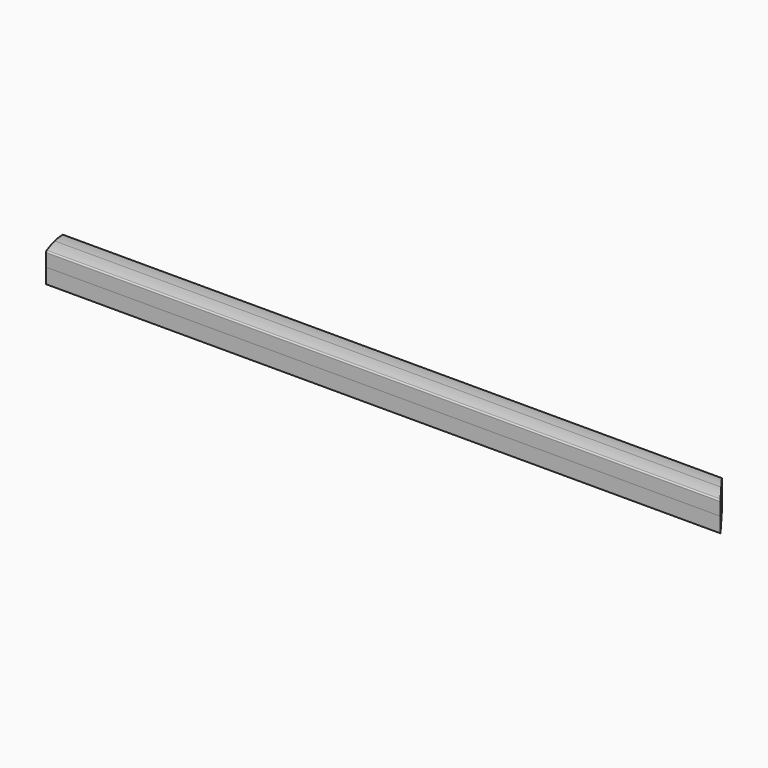
from build123d import *

# Parameters (mm, degrees)
F2_DEPTH      = 1000
F4_DEPTH      = 1000
F8_DEPTH      = 10.001
F8_DEPTH_BACK = 10.001


with BuildPart() as f2:
    # F1 (on Right) → F2 (new body)
    with BuildSketch(Plane.YZ):
        with BuildLine():
            Line((0, -9), (0, -10))
            Line((0, -10), (10, -10))
            Line((10, -10), (10, -0.2))
            Line((10, -0.2), (9, -0.2))
            ThreePointArc((9, -0.2), (8.5, -0.7), (9, -1.2))
            ThreePointArc((9, -1.2), (9.5, -1.7), (9, -2.2))
            Line((9, -2.2), (9, -9))
            Line((9, -9), (0, -9))
        make_face()
    extrude(amount=F2_DEPTH)

    # F5: F2 across plane


with BuildPart() as f4:
    # F3 (on Right) → F4 (new body)
    with BuildSketch(Plane.YZ):
        with BuildLine():
            Line((9, -0.2), (10, -0.2))
            Line((10, -0.2), (10, 8.1663783152))
            ThreePointArc((10, 8.1663783152), (9.7693092582, 8.8052548802), (9.1836734694, 9.1493656277))
            ThreePointArc((9.1836734694, 9.1493656277), (4.6114920912, 9.7868872364), (0, 10))
            Line((0, 10), (0, 9))
            ThreePointArc((0, 9), (4.5192622493, 8.7911494917), (9, 8.1663783152))
            Line((9, 8.1663783152), (9, 0.8))
            ThreePointArc((9, 0.8), (7.5, -0.7), (9, -2.2))
            ThreePointArc((9, -2.2), (9.5, -1.7), (9, -1.2))
            ThreePointArc((9, -1.2), (8.5, -0.7), (9, -0.2))
        make_face()
    extrude(amount=F4_DEPTH)

    # F6: F4 across plane


with BuildPart() as f2_1:
    add(f2.part)
    add(f2.part.mirror(Plane.XZ))


with BuildPart() as f4_1:
    add(f4.part)
    add(f4.part.mirror(Plane.XZ))


with BuildPart() as f8_tool:
    # F7 (on Top) → F8 (new body, two sides)
    with BuildSketch(Plane.XY) as f8_sk:
        Polygon((0, 10), (0, 0), (0, -10), (4.8015751816, -10), align=None)
        Polygon((444.8015751816, 10), (429.7304941795, 10), (444.8015751816, -10), (1016.9613361359, -10), (1016.9613361359, 10), align=None)
    extrude(amount=F8_DEPTH)
    extrude(f8_sk.sketch, amount=-F8_DEPTH_BACK)


with BuildPart() as f2_2:
    add(f2_1.part)

    # F8: cut by f8_tool
    add(f8_tool.part, mode=Mode.SUBTRACT)


with BuildPart() as f4_2:
    add(f4_1.part)

    # F8: cut by f8_tool
    add(f8_tool.part, mode=Mode.SUBTRACT)


solid = Compound([f2_2.part, f4_2.part])
